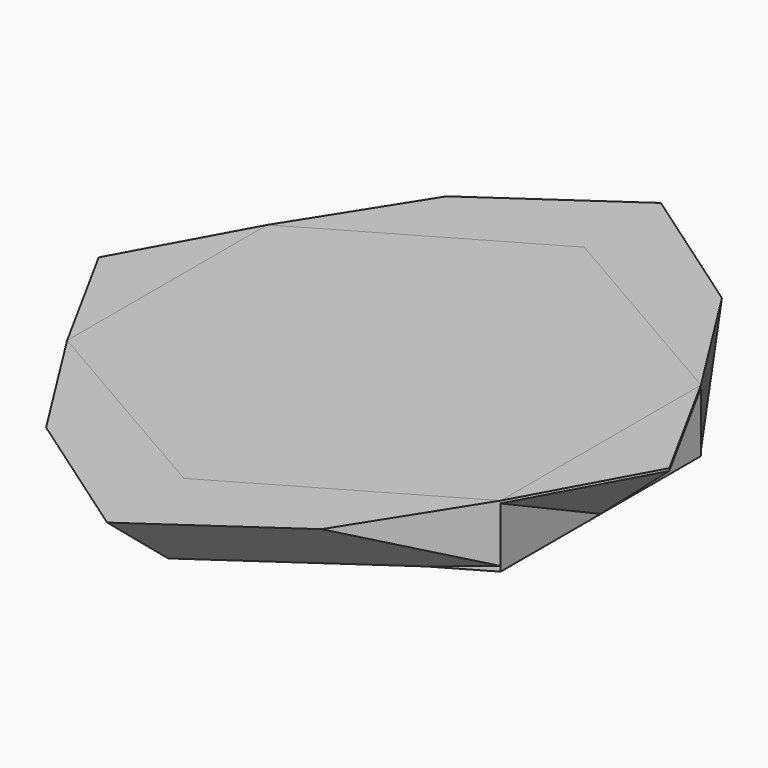
from build123d import *

# Parameters (mm, degrees)
F2_DEPTH  = 25
F3_SIZE   = 24.99999
F3_2_SIZE = 24.99999
F4_SIZE   = 24
F4_2_SIZE = 24


# Not quite as in the source:
# - a fillet or chamfer is up to 0.001 mm smaller than in the source, because OpenCascade refuses the exact size
# - a feature names something its author has since deleted; it is built from what else it names


with BuildPart() as f2:
    # F1 (on face) → F2 (new body)
    with BuildSketch(Plane.XY):
        Polygon((-86.6025403784, -50), (0, -100), (86.6025403784, -50), (86.6025403784, 50), (0, 100), (-86.6025403784, 50), align=None)
    extrude(amount=F2_DEPTH)


with BuildPart() as f2b:
    # F0 (on Top) → F2, piece 2 (new body)
    with BuildSketch(Plane.XY):
        Polygon((0, 100), (86.6025403784, 50), (55, 100), align=None)
        Polygon((-86.6025403784, 50), (0, 100), (-55, 100), align=None)
        Polygon((-55, 100), (0, 100), (55, 100), (0, 138.2622529394), align=None)
    extrude(amount=F2_DEPTH)

    # F3 (size 25 in the source; OpenCascade refuses exactly that, so slightly less here)
    f3_edges = [f2b.edges().sort_by_distance(p)[0] for p in [
        (-27.5, 119.131126, 0),
        (27.5, 119.131126, 0),
    ]]
    chamfer(f3_edges, length=F3_SIZE)


with BuildPart() as f2c:
    # F0 (on Top) → F2, piece 3 (new body)
    with BuildSketch(Plane.XY):
        Polygon((-113.9704047453, 0), (-86.6025403784, -50), (-86.6025403784, 50), align=None)
    extrude(amount=F2_DEPTH)

    # F4
    f4_edges = [f2c.edges().sort_by_distance(p)[0] for p in [
        (-100.286473, 25, 0),
        (-100.286473, -25, 0),
    ]]
    chamfer(f4_edges, length=F4_SIZE)


with BuildPart() as f2d:
    # F0 (on Top) → F2, piece 4 (new body)
    with BuildSketch(Plane.XY):
        Polygon((-55, -100), (0, -100), (-86.6025403784, -50), align=None)
        Polygon((55, -100), (86.6025403784, -50), (0, -100), align=None)
        Polygon((55, -100), (0, -100), (-55, -100), (0, -138.2622529394), align=None)
    extrude(amount=F2_DEPTH)

    # F3#2 (size 25 in the source; OpenCascade refuses exactly that, so slightly less here)
    f3_2_edges = [f2d.edges().sort_by_distance(p)[0] for p in [
        (-27.5, -119.131126, 0),
        (27.5, -119.131126, 0),
    ]]
    chamfer(f3_2_edges, length=F3_2_SIZE)


with BuildPart() as f2e:
    # F0 (on Top) → F2, piece 5 (new body)
    with BuildSketch(Plane.XY):
        Polygon((86.6025403784, 50), (86.6025403784, -50), (113.9704047453, 0), align=None)
    extrude(amount=F2_DEPTH)

    # F4#2
    f4_2_edges = [f2e.edges().sort_by_distance(p)[0] for p in [
        (100.286473, -25, 0),
        (100.286473, 25, 0),
    ]]
    chamfer(f4_2_edges, length=F4_2_SIZE)


solid = Compound([f2.part, f2b.part, f2c.part, f2d.part, f2e.part])
